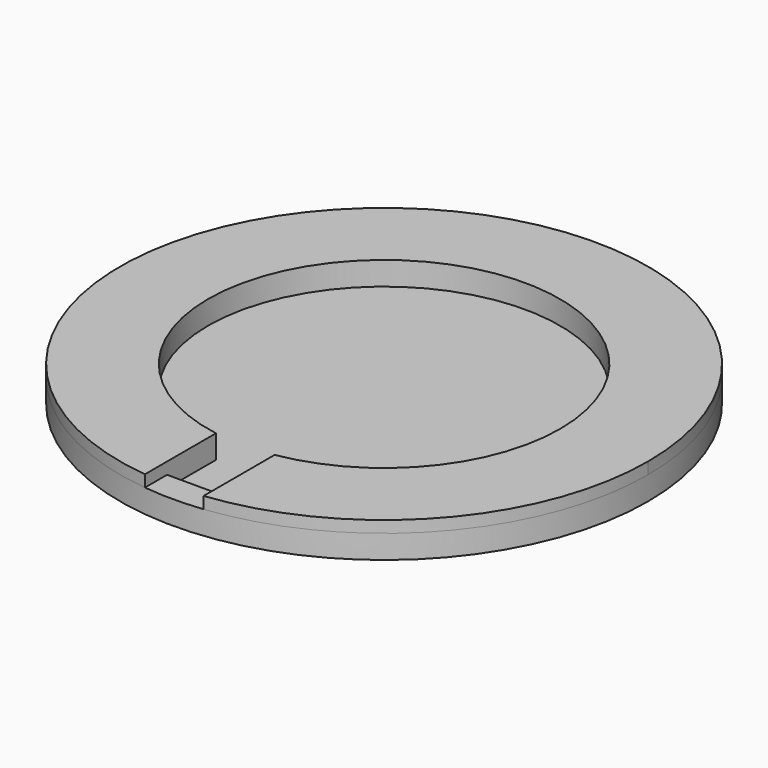
from build123d import *

# Parameters (mm, degrees)
F1_R     = 57.15
F2_DEPTH = 2.54
F3_R     = 57.15
F4_DEPTH = 2.54
F6_DEPTH = 2.54


with BuildPart() as f2:
    # F1 (on Top) → F2 (new body)
    with BuildSketch(Plane.XY):
        Circle(F1_R)
    extrude(amount=F2_DEPTH)

    # F3 (on face) → F4 (join)
    with BuildSketch(Plane.XY.offset(2.54)):
        Circle(F3_R)
        with BuildLine():
            ThreePointArc((-6.35, -37.567107), (0, 38.1), (6.35, -37.567107))
            Line((6.35, -37.567107), (6.35, -50.8))
            Line((6.35, -50.8), (-6.35, -50.8))
            Line((-6.35, -50.8), (-6.35, -37.567107))
        make_face(mode=Mode.SUBTRACT)
    extrude(amount=F4_DEPTH)

    # F5 (on face) → F6 (join)
    with BuildSketch(Plane.XY.offset(5.08)):
        with BuildLine():
            Line((6.35, -50.8), (6.35, -56.796127))
            ThreePointArc((6.35, -56.796127), (42.597095, -38.1), (57.15, 0))
            ThreePointArc((57.15, 0), (-38.1, 42.597095), (-6.35, -56.796127))
            Line((-6.35, -56.796127), (-6.35, -50.8))
            Line((-6.35, -50.8), (-6.35, -37.567107))
            ThreePointArc((-6.35, -37.567107), (0, 38.1), (6.35, -37.567107))
            Line((6.35, -37.567107), (6.35, -50.8))
        make_face()
    extrude(amount=F6_DEPTH)


solid = f2.part
